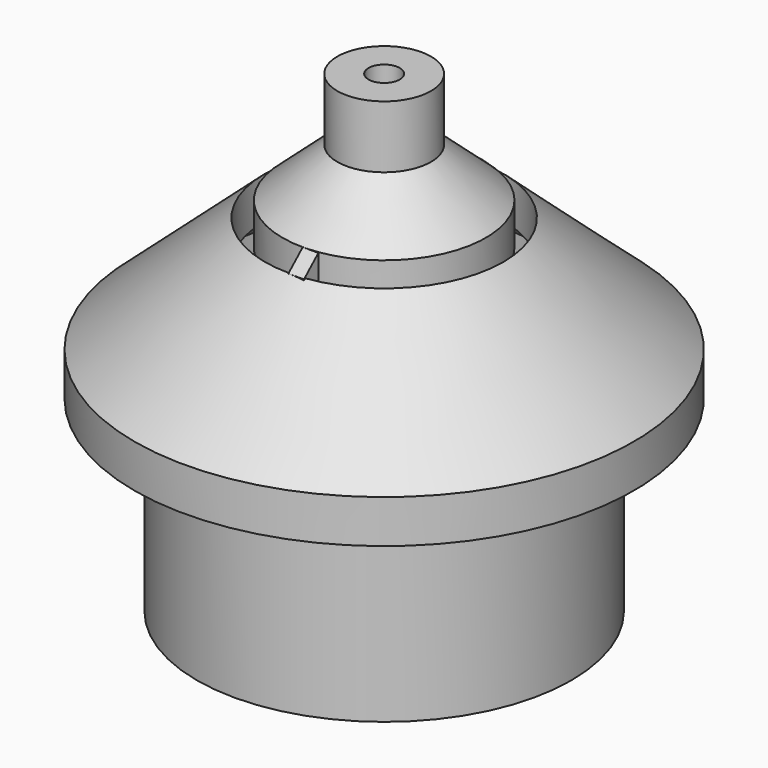
from build123d import *

# Parameters (mm, degrees)
F3_DEPTH = 0.5


# Not quite as in the source:
# - a pattern or mirror of a feature is missing from the dataset's text; its kind, count and spacing are read off the source's solid


with BuildPart() as f1:
    # F0 (on Front) → F1 (revolve)
    with BuildSketch(Plane.XZ):
        Polygon((-6, 6), (-6, 0), (-5, 0), (-5, 8.7112633561), (-3.8233768799, 9.7571505739), (-3.8233768799, 11.0951055271), (-8, 7.3825516426), (-8, 6), align=None)
    revolve(axis=Axis((0, 0, 1.3750899837), (0, 0, 1)))

    # F2 (on Right) → F3 (join)
    with BuildSketch(Plane.YZ):
        Polygon((-3.261596497, 10.5184856802), (-3.261596497, 11.5944658675), (-3.8373894771, 11.0826498851), (-3.8373894771, 10.0066696978), align=None)
    f3 = extrude(amount=F3_DEPTH)

    # F3_copies: F3 across plane
    add(f3.mirror(Plane.ZX))


with BuildPart() as f1b:
    # F0 (on Front) → F1, piece 2 (revolve)
    with BuildSketch(Plane.XZ):
        Polygon((-1.5, 15.1603294204), (-1.5, 13.1603294204), (-3.261596497, 11.5944658675), (-3.261596497, 10.2565109143), (-2.5, 10.9334855783), (-2.5, 0), (-0.5, 0), (-0.5, 12.7112633561), (-0.5, 15.1603294204), align=None)
    revolve(axis=Axis((0, 0, 1.3750899837), (0, 0, 1)))


solid = Compound([f1.part, f1b.part])
